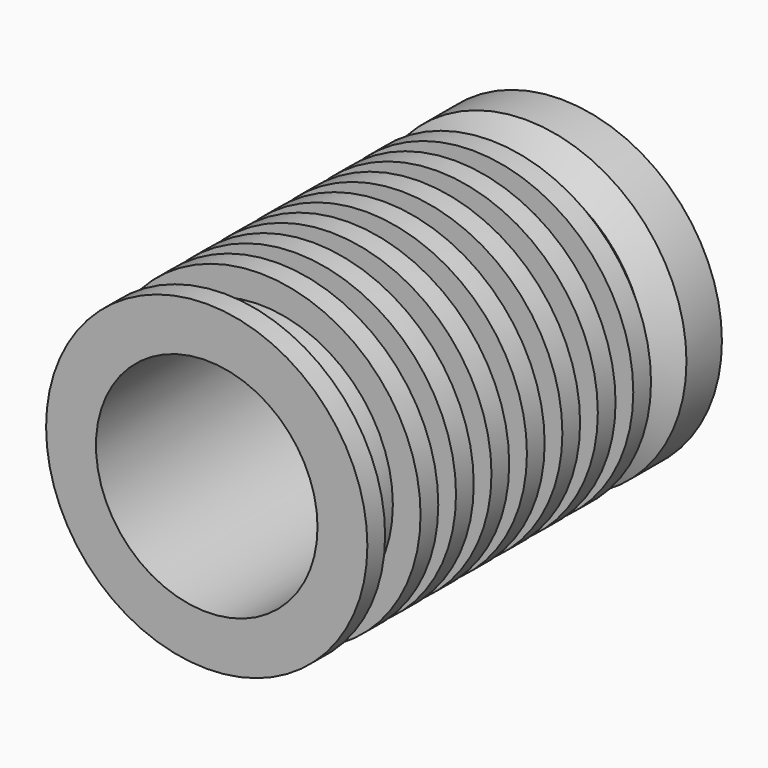
from build123d import *

# Parameters (mm, degrees)
F1_START     = -88.9
F0_R         = 18.415
F0_R_2       = 12.7
F1_DEPTH     = 12.7
F2_START     = -83.82
F2_DEPTH     = 2.54
F3_START     = -78.74
F3_DEPTH     = 2.54
F4_START     = -73.66
F4_DEPTH     = 2.54
F5_START     = -68.58
F5_DEPTH     = 2.54
F6_START     = -63.5
F6_DEPTH     = 2.54
F7_START     = -58.42
F7_DEPTH     = 2.54
F8_DEPTH     = 55.88
F9_R         = 15.24
F9_R_2       = 12.7
F10_DEPTH    = 101.6
F11_S5_R     = 15.24
F11_T6_DEPTH = 28
F12_S5_R     = 15.24
F12_T6_DEPTH = 53
F13_START    = -88.9
F13_DEPTH    = 2.54
F14_DEPTH    = 50.8


# Not quite as in the source:
# - a fillet or chamfer that OpenCascade refuses, or shapes differently, is made with other operations: its cross-section is extruded or revolved along the edge and cut away or added


with BuildPart() as f1:
    # F0 (on Front) → F1 (new body)
    with BuildSketch(Plane.XZ.offset(F1_START)):
        Circle(F0_R)
        Circle(F0_R_2, mode=Mode.SUBTRACT)
    extrude(amount=-F1_DEPTH)



with BuildPart() as f2:
    # F0 (on Front) → F2 (new body)
    with BuildSketch(Plane.XZ.offset(F2_START)):
        Circle(F0_R)
        Circle(F0_R_2, mode=Mode.SUBTRACT)
    extrude(amount=-F2_DEPTH)


with BuildPart() as f3:
    # F0 (on Front) → F3 (new body)
    with BuildSketch(Plane.XZ.offset(F3_START)):
        Circle(F0_R)
        Circle(F0_R_2, mode=Mode.SUBTRACT)
    extrude(amount=-F3_DEPTH)


with BuildPart() as f4:
    # F0 (on Front) → F4 (new body)
    with BuildSketch(Plane.XZ.offset(F4_START)):
        Circle(F0_R)
        Circle(F0_R_2, mode=Mode.SUBTRACT)
    extrude(amount=-F4_DEPTH)


with BuildPart() as f5:
    # F0 (on Front) → F5 (new body)
    with BuildSketch(Plane.XZ.offset(F5_START)):
        Circle(F0_R)
        Circle(F0_R_2, mode=Mode.SUBTRACT)
    extrude(amount=-F5_DEPTH)


with BuildPart() as f6:
    # F0 (on Front) → F6 (new body)
    with BuildSketch(Plane.XZ.offset(F6_START)):
        Circle(F0_R)
        Circle(F0_R_2, mode=Mode.SUBTRACT)
    extrude(amount=-F6_DEPTH)


with BuildPart() as f7:
    # F0 (on Front) → F7 (new body)
    with BuildSketch(Plane.XZ.offset(F7_START)):
        Circle(F0_R)
        Circle(F0_R_2, mode=Mode.SUBTRACT)
    extrude(amount=-F7_DEPTH)


with BuildPart() as f8:
    # F0 (on Front) → F8 (new body)
    with BuildSketch(Plane.XZ):
        Circle(F0_R)
        Circle(F0_R_2, mode=Mode.SUBTRACT)
    extrude(amount=-F8_DEPTH)


with BuildPart() as f1_1:
    add(f1.part)

    add(f2.part)  # F10 merges F2

    add(f3.part)  # F10 merges F3

    add(f4.part)  # F10 merges F4

    add(f5.part)  # F10 merges F5

    add(f6.part)  # F10 merges F6

    add(f7.part)  # F10 merges F7

    add(f8.part)  # F10 merges F8
    # F9 (on Front) → F10 (join)
    with BuildSketch(Plane.XZ):
        Circle(F9_R)
        Circle(F9_R_2, mode=Mode.SUBTRACT)
    extrude(amount=-F10_DEPTH)

    # F11: chamfer of 2.54 x 3.81 on 1 edges, made by hand


with BuildPart() as f11_tool2:
    # F11_s3 → F11_t4 (revolve)
    with BuildSketch(Plane.XY):
        Polygon((18.415, 53.34), (14.605, 55.88), (18.415, 55.88), align=None)
    revolve(axis=Axis((0, 55.88, 0), (0, -1, 0)))

    # F11_s5 → F11_t6 (cut, symmetric)
    with BuildSketch(Plane.XZ.offset(-54.6)):
        Circle(F11_S5_R)
    extrude(amount=F11_T6_DEPTH, both=True, mode=Mode.SUBTRACT)


with BuildPart() as f1_2:
    add(f1_1.part)

    # F11_t1: cut F11_tool2
    add(f11_tool2.part, mode=Mode.SUBTRACT)

    # F12: chamfer of 12.7 x 7.62 on 1 edges, made by hand


with BuildPart() as f12_tool2:
    # F12_s3 → F12_t4 (revolve)
    with BuildSketch(Plane.XY):
        with BuildLine():
            Line((5.2793935937, 88.6386361562), (18.8506064063, 96.7813638438))
            Line((18.8506064063, 96.7813638438), (19.1046064063, 96.7813638438))
            ThreePointArc((19.1046064063, 96.7813638438), (18.669, 92.8406819219), (18.669, 88.9))
            Line((18.669, 88.9), (18.415, 88.646))
            ThreePointArc((18.415, 88.646), (11.8471967969, 88.646), (5.2793935937, 88.3846361562))
            Line((5.2793935937, 88.3846361562), (5.2793935937, 88.6386361562))
        make_face()
    revolve(axis=Axis((0, 88.9, 0), (0, -1, 0)))

    # F12_s5 → F12_t6 (cut, symmetric)
    with BuildSketch(Plane.XZ.offset(-90.9)):
        Circle(F12_S5_R)
    extrude(amount=F12_T6_DEPTH, both=True, mode=Mode.SUBTRACT)


with BuildPart() as f1_3:
    add(f1_2.part)

    # F12_t1: cut F12_tool2
    add(f12_tool2.part, mode=Mode.SUBTRACT)

    # F0 (on Front) → F13 (join)
    with BuildSketch(Plane.XZ.offset(F13_START)):
        Circle(F0_R)
        Circle(F0_R_2, mode=Mode.SUBTRACT)
    extrude(amount=-F13_DEPTH)

    # F0 (on Front) → F14 (cut)
    with BuildSketch(Plane.XZ):
        Circle(F0_R)
        Circle(F0_R_2, mode=Mode.SUBTRACT)
    extrude(amount=-F14_DEPTH, mode=Mode.SUBTRACT)


solid = f1_3.part
